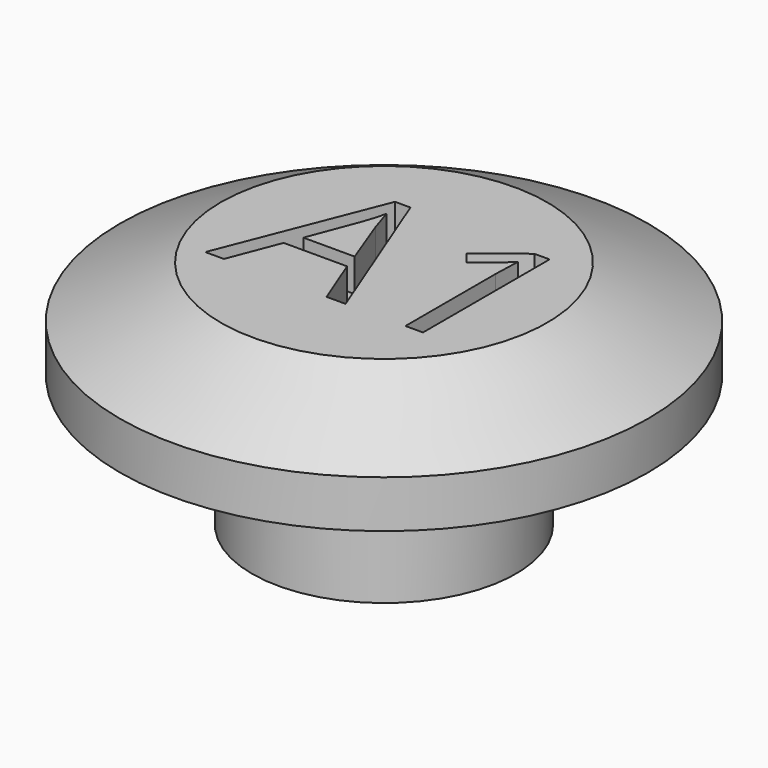
from build123d import *

# Parameters (mm, degrees)
F2_TEXT_SIZE = 170.5611745516
F3_DEPTH     = 25.4


# Not quite as in the source:
# - Text() gives the source's letters only with a copy of the font that has no kerning and outlines rounded to 1/6400 em; it was checked with that copy


with BuildPart() as f1:
    # F0 (on Front) → F1 (revolve)
    with BuildSketch(Plane.XZ):
        Polygon((-101.6, 0), (0, 0), (0, 177.8), (-203.2, 177.8), (-203.2, 101.6), (-101.6, 101.6), align=None)
    revolve(axis=Axis((0, 0, -2.0734842505), (0, 0, -1)))

    # F2 (on face) → F3 (cut)
    with BuildSketch(Plane.XY.offset(177.8)):
        with Locations((-92.2999605536, -56.4873867843)):
            Text('A1', F2_TEXT_SIZE, font='Open Sans', text_align=(TextAlign.LEFT, TextAlign.BOTTOM))
    extrude(amount=-F3_DEPTH, mode=Mode.SUBTRACT)

    # F4 (on Front) → F5 (revolve, cut)
    with BuildSketch(Plane.XZ):
        Polygon((-215.3274565935, 184.3061447144), (-203.7725448608, 137.7741843462), (-123.8249987364, 178.6848306656), align=None)
    revolve(axis=Axis((0, 0, 69.355532527), (0, 0, 1)), mode=Mode.SUBTRACT)


solid = f1.part
